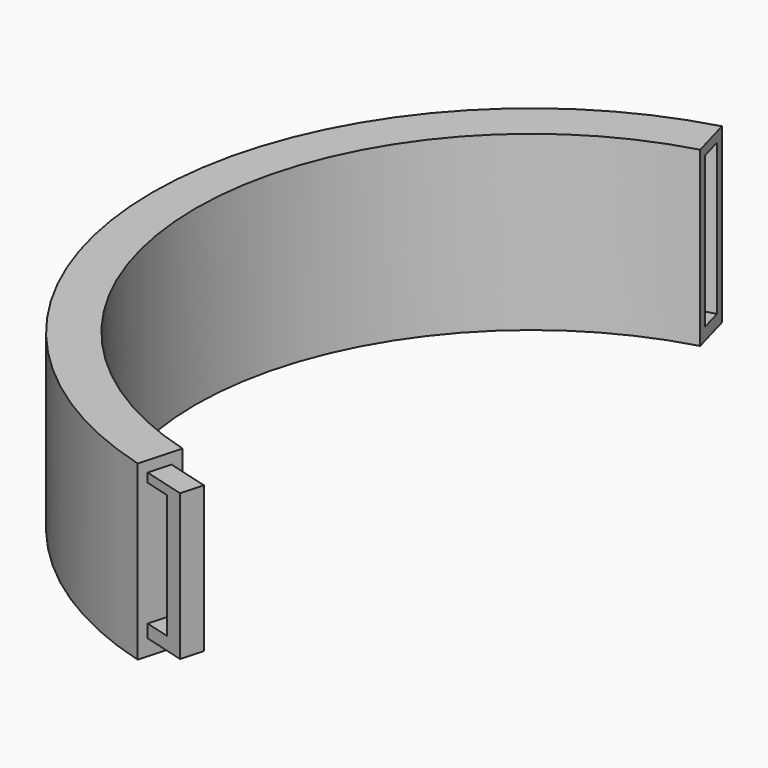
from build123d import *

# Parameters (mm, degrees)
F1_DEPTH  = 20
F2_W      = 2.6613399386
F2_H      = 1.0413937271
F2_H_2    = 1.5042340383
F3_DEPTH  = 3
F5_DEPTH  = 2
F6_W      = 2.6971405605
F6_H      = 17.4564992776
F7_DEPTH  = 5
F9_W      = 1.6222847626
F9_H      = 16.6863657068
F10_DEPTH = 4.8


# Not quite as in the source:
# - ends of sketch curves that miss each other by under 0.0002 mm in the source are joined


with BuildPart() as f1:
    # F0 (on Top) → F1 (new body)
    with BuildSketch(Plane.XY):
        with BuildLine():
            ThreePointArc((0, -74.9042034149), (-28.4520233491, -37.4521017075), (0, 0))
            Line((0, 0), (-1.3406298741, 4.8169190701))
            ThreePointArc((-1.3406298741, 4.8169190701), (-33.4520231279, -37.4521017075), (-1.3406298741, -79.7211224851))
            Line((-1.3406298741, -79.7211224851), (0, -74.9042034149))
        make_face()
    extrude(amount=F1_DEPTH)

    # F2 (on face) → F3 (join)
    with BuildSketch(Plane(origin=(19.3483734862, -5.3849788907, 0), x_dir=(0.2681259867, 0.9633838567, 0), z_dir=(0.9633838567, -0.2681259867, 0))):
        with Locations((-74.7193582356, 18.2154309005)):
            Rectangle(F2_W, F2_H)
        with Locations((-74.7193582356, 2.5945375673)):
            Rectangle(F2_W, F2_H_2)
    extrude(amount=F3_DEPTH)

    # F4 (on face) → F5 (join)
    with BuildSketch(Plane(origin=(22.2385250561, -6.1893568507, 0), x_dir=(0.2681259867, 0.9633838567, 0), z_dir=(0.9633838567, -0.2681259867, 0))):
        Polygon((-73.3886882663, 17.6947340369), (-76.0500282049, 17.6947340369), (-76.0500282049, 1.8424974987), (-73.3886659145, 1.8424974987), align=None)
        Polygon((-73.3886659145, 18.736127764), (-76.0500282049, 18.736127764), (-76.0500282049, 17.6947340369), (-73.3886882663, 17.6947340369), align=None)
    extrude(amount=F5_DEPTH)

    # F6 (on face) → F7 (cut)
    with BuildSketch(Plane(origin=(0, 0, 0), x_dir=(-0.2681259867, 0.9633838567, 0), z_dir=(0.9633838567, 0.2681259867, 0))):
        with Locations((2.4999994203, 10.1498414879)):
            Rectangle(F6_W, F6_H)
    extrude(amount=-F7_DEPTH, mode=Mode.SUBTRACT)

    # F9 (on offset) → F10 (cut)
    with BuildSketch(Plane.XZ.offset(-4.7)):
        with Locations((-6.0561252758, 9.9340636516)):
            Rectangle(F9_W, F9_H)
    extrude(amount=F10_DEPTH, mode=Mode.SUBTRACT)


solid = f1.part
